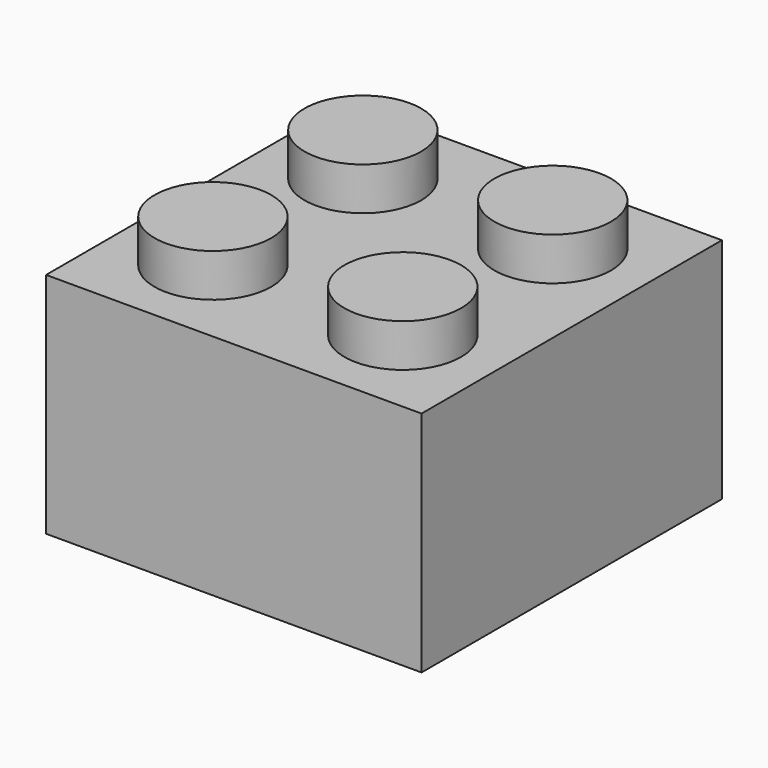
from build123d import *

# Parameters (mm, degrees)
F0_W     = 15.7734
F0_H     = 15.7734
F1_DEPTH = 9.5758
F2_R     = 2.4511
F3_DEPTH = 1.8034
F5_W     = 13.1826
F5_H     = 13.1826
F5_R     = 3.1299195118
F6_DEPTH = 8.3566


# Not quite as in the source:
# - a feature names something its author has since deleted; it is built from what else it names


with BuildPart() as f1:
    # F0 (on Top) → F1 (new body)
    with BuildSketch(Plane.XY):
        Rectangle(F0_W, F0_H)
    extrude(amount=F1_DEPTH)

    # F2 (on face) → F3 (join)
    with BuildSketch(Plane.XY.offset(9.5758)):
        with Locations((-4.0386, -3.937)):
            Circle(F2_R)
        with Locations((3.937, -3.937)):
            Circle(F2_R)
        with Locations((3.937, 3.937)):
            Circle(F2_R)
        with Locations((-4.0386, 3.937)):
            Circle(F2_R)
    extrude(amount=F3_DEPTH)

    # F5 (on face) → F6 (cut)
    with BuildSketch(Plane(origin=(0, 0, 0), x_dir=(1, 0, 0), z_dir=(0, 0, -1))):
        Rectangle(F5_W, F5_H)
        Circle(F5_R, mode=Mode.SUBTRACT)
    extrude(amount=-F6_DEPTH, mode=Mode.SUBTRACT)


solid = f1.part
